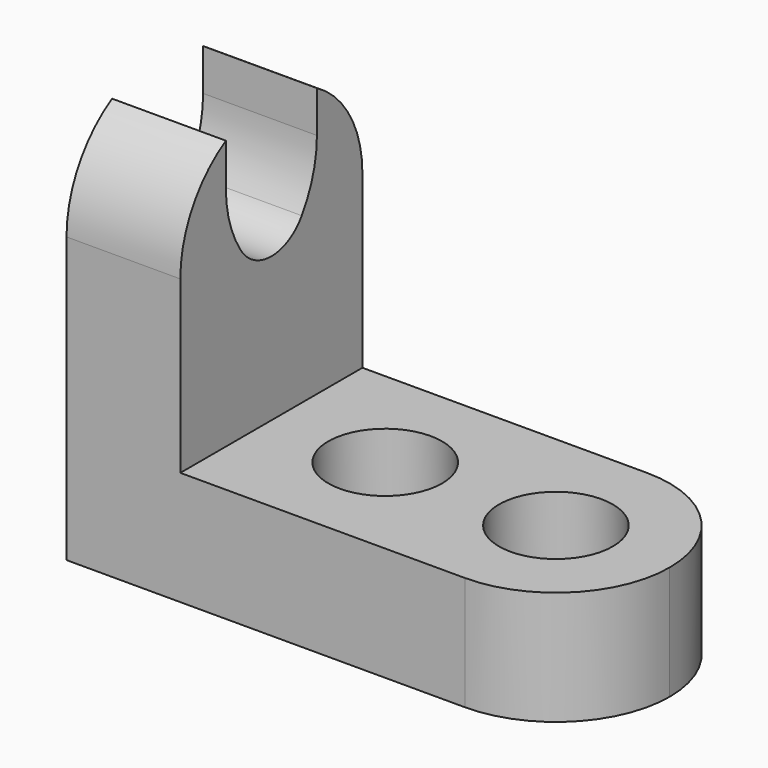
from build123d import *

# Parameters (mm, degrees)
F1_DEPTH    = 25.4
F2_R        = 12.7
F3_R        = 12.69999
F4_R        = 12.7
F5_T1_DEPTH = 76.2
F6_W        = 12.7
F6_H        = 17.3485226281
F7_DEPTH    = 25.4
F9_T1_DEPTH = 12.7
F10_R       = 5.08
F11_R       = 6.35
F12_DEPTH   = 12.7


# Not quite as in the source:
# - a fillet or chamfer that OpenCascade refuses, or shapes differently, is made with other operations: its cross-section is extruded or revolved along the edge and cut away or added
# - a fillet or chamfer is up to 0.001 mm smaller than in the source, because OpenCascade refuses the exact size
# - a feature of the source that left no trace in its solid (it failed there, or was rolled back) is left out


with BuildPart() as f1:
    # F0 (on Front) → F1 (new body)
    with BuildSketch(Plane.XZ):
        Polygon((0, 44.45), (0, 0), (57.15, 0), (57.15, 12.7), (12.7, 12.7), (12.7, 44.45), align=None)
    extrude(amount=F1_DEPTH)

    # F2
    f2_edges = [f1.edges().sort_by_distance(p)[0] for p in [
        (57.15, -25.4, 6.35),
    ]]
    fillet(f2_edges, radius=F2_R)

    # F3 (radius 12.7 in the source; OpenCascade refuses exactly that, so slightly less here)
    f3_edges = [f1.edges().sort_by_distance(p)[0] for p in [
        (57.15, 0, 6.35),
    ]]
    fillet(f3_edges, radius=F3_R)

    # F4
    f4_edges = [f1.edges().sort_by_distance(p)[0] for p in [
        (6.35, -25.4, 44.45),
    ]]
    fillet(f4_edges, radius=F4_R)

    # F5: fillet of radius 12.7 on 1 edges, made by hand

    # F5_s2 → F5_t1 (cut)
    with BuildSketch(Plane.YZ.offset(-31.75)):
        with BuildLine():
            ThreePointArc((-12.7, 44.45), (-3.7197438789, 40.7302561211), (0, 31.75))
            Line((0, 31.75), (0, 44.45))
            Line((0, 44.45), (-12.7, 44.45))
        make_face()
    extrude(amount=F5_T1_DEPTH, mode=Mode.SUBTRACT)

    # F6 (on face) → F7 (cut)
    with BuildSketch(Plane.YZ.offset(12.7)):
        with BuildLine():
            ThreePointArc((-12.7, 44.45), (-15.9870018728, 44.0172579939), (-19.05, 42.7485226281))
            Line((-19.05, 42.7485226281), (-6.35, 42.7485226281))
            ThreePointArc((-6.35, 42.7485226281), (-9.4129981272, 44.0172579939), (-12.7, 44.45))
        make_face()
        with Locations((-12.7, 34.074261314)):
            Rectangle(F6_W, F6_H)
    extrude(amount=-F7_DEPTH, mode=Mode.SUBTRACT)

    # F9: fillet of radius 12.7 on 2 edges, made by hand

    # F9_s2 → F9_t1 (join)
    with BuildSketch(Plane.YZ):
        with BuildLine():
            ThreePointArc((-19.05, 38.1), (-15.3302561211, 29.1197438789), (-6.35, 25.4))
            Line((-6.35, 25.4), (-19.05, 25.4))
            Line((-19.05, 25.4), (-19.05, 38.1))
        make_face()
        with BuildLine():
            ThreePointArc((-19.05, 25.4), (-10.0697438789, 29.1197438789), (-6.35, 38.1))
            Line((-6.35, 38.1), (-6.35, 25.4))
            Line((-6.35, 25.4), (-19.05, 25.4))
        make_face()
    extrude(amount=F9_T1_DEPTH)

    # F10
    f10_edges = [f1.edges().sort_by_distance(p)[0] for p in [
        (6.35, -12.7, 27.101477),
    ]]
    fillet(f10_edges, radius=F10_R)

    # F11 (on face) → F12 (cut)
    with BuildSketch(Plane.XY.offset(12.7)):
        with Locations((25.4, -12.7)):
            Circle(F11_R)
        with Locations((44.45, -12.7)):
            Circle(F11_R)
    extrude(amount=-F12_DEPTH, mode=Mode.SUBTRACT)


solid = f1.part
